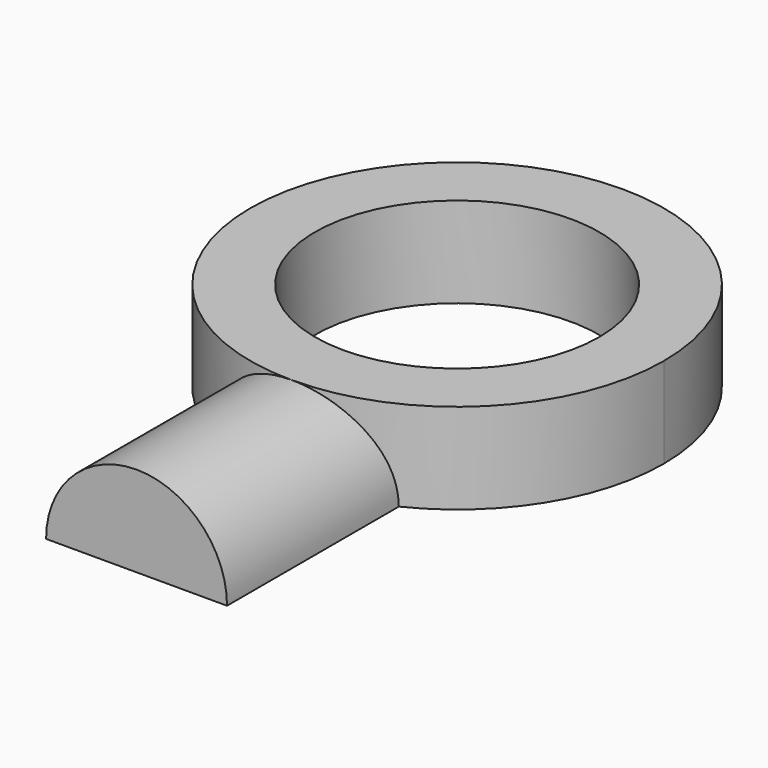
from build123d import *
from build123d import SkipClean  # not in build123d's __all__

# Parameters (mm, degrees)
F1_DEPTH = 20
F2_R     = 16
F2_R_2   = 11
F3_DEPTH = 7


with BuildPart() as f1:
    # F0 (on Front) → F1 (new body)
    with BuildSketch(Plane.XZ):
        with BuildLine():
            Line((-2, 0), (0, 0))
            Line((0, 0), (10, 0))
            Line((10, 0), (12, 0))
            ThreePointArc((12, 0), (5, 7), (-2, 0))
        make_face()
    extrude(amount=F1_DEPTH)

    # F2 (on Top) → F3 (join)
    with BuildSketch(Plane.XY):
        with Locations((5, 11)):
            Circle(F2_R)
        with Locations((5, 11)):
            Circle(F2_R_2, mode=Mode.SUBTRACT)
    with SkipClean():  # cleaning this boolean's faces spoils the solid; the shape is the same uncleaned
        extrude(amount=F3_DEPTH)


solid = f1.part
